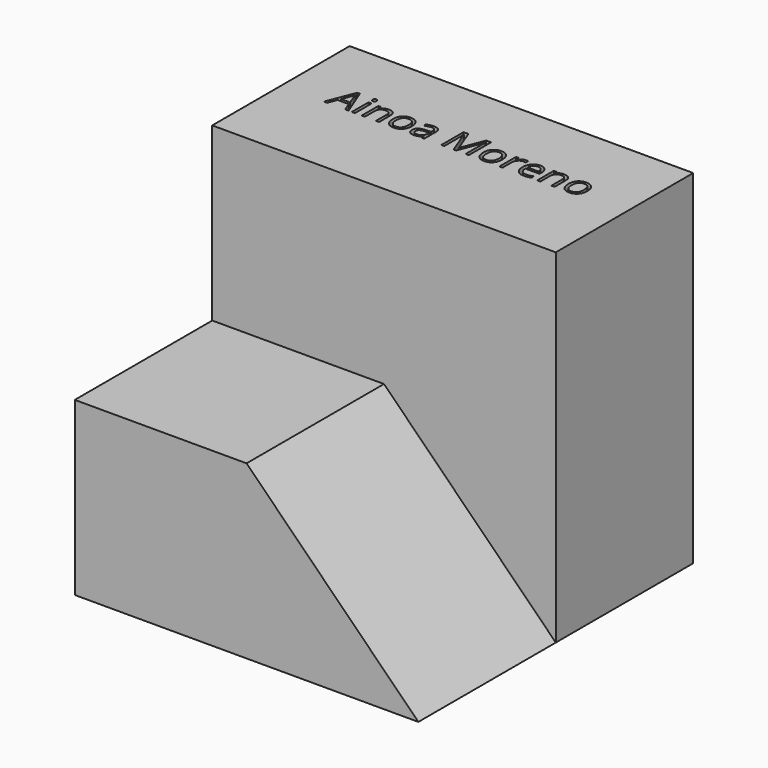
from build123d import *

# Parameters (mm, degrees)
F0_W         = 40
F0_H         = 40
F1_DEPTH     = 20
F3_DEPTH     = 20
F4_TEXT_SIZE = 4.5302250956
F5_DEPTH     = 2


# Not quite as in the source:
# - Text() gives the source's letters only with a copy of the font that has no kerning and outlines rounded to 1/6400 em; it was checked with that copy


with BuildPart() as f1:
    # F0 (on Front) → F1 (new body)
    with BuildSketch(Plane.XZ):
        with Locations((20, 20)):
            Rectangle(F0_W, F0_H)
    extrude(amount=F1_DEPTH)

    # F2 (on face) → F3 (join)
    with BuildSketch(Plane.XZ.offset(20)):
        Polygon((0, 20), (0, 0), (40, 0), (20, 20), align=None)
    extrude(amount=F3_DEPTH)

    # F4 (on face) → F5 (cut)
    with BuildSketch(Plane.XY.offset(40)):
        with Locations((5, -10)):
            Text('Ainoa Moreno', F4_TEXT_SIZE, font='Open Sans', text_align=(TextAlign.LEFT, TextAlign.BOTTOM))
    extrude(amount=-F5_DEPTH, mode=Mode.SUBTRACT)


solid = f1.part
